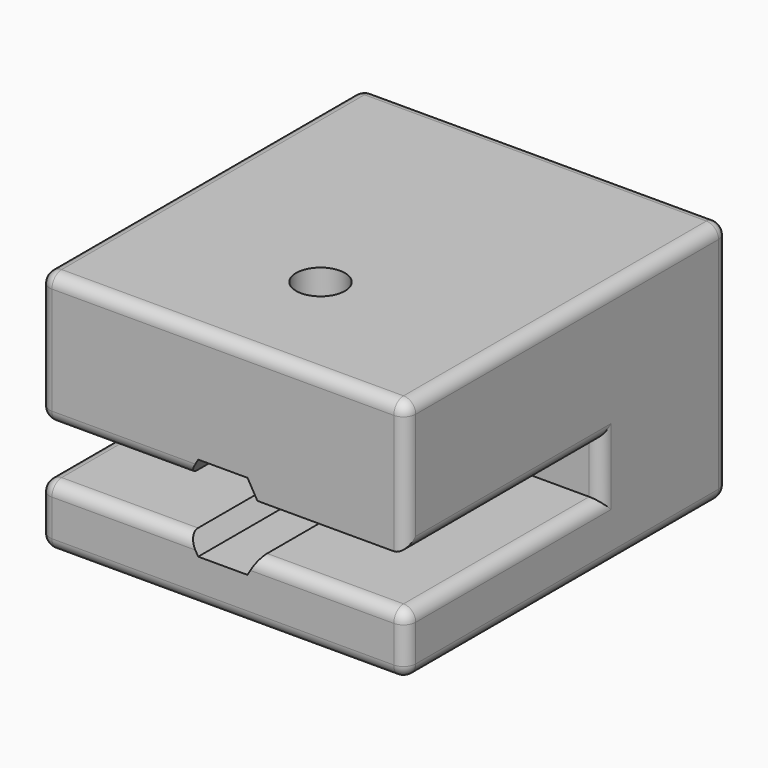
from build123d import *

# Parameters (mm, degrees)
F0_W          = 30
F0_H          = 33
F1_DEPTH      = 20
F2_W          = 20
F2_H          = 4.2
F3_DEPTH      = 30.001
F4_R          = 2
F5_DEPTH      = 5
F5_DEPTH_BACK = 20.001
F6_DEPTH      = 13.001
F7_R          = 2
F8_DEPTH      = 10.801
F9_DEPTH      = 3.5
F10_R         = 1


with BuildPart() as f1:
    # F0 (on Top) → F1 (new body)
    with BuildSketch(Plane.XY):
        Rectangle(F0_W, F0_H)
    extrude(amount=F1_DEPTH)

    # F2 (on face) → F3 (cut, through all)
    with BuildSketch(Plane.YZ.offset(15)):
        with Locations((-6.5, 7.1)):
            Rectangle(F2_W, F2_H)
    extrude(amount=-F3_DEPTH, mode=Mode.SUBTRACT)

    # F4 (on face) → F5 (cut, two sides)
    with BuildSketch(Plane.XZ.offset(-3.5)) as f5_sk:
        Polygon((-2.829016319, 9.2), (2.829016319, 9.2), (2.0207259422, 10.6), (-2.0207259422, 10.6), align=None)
        Polygon((-2.829016319, 5), (2.829016319, 5), (4.0414518843, 7.1), (2.829016319, 9.2), (-2.829016319, 9.2), (-4.0414518843, 7.1), align=None)
        with Locations((0, 7.1)):
            Circle(F4_R, mode=Mode.SUBTRACT)
        Polygon((-2.0207259422, 3.6), (2.0207259422, 3.6), (2.829016319, 5), (-2.829016319, 5), align=None)
    extrude(amount=-F5_DEPTH, mode=Mode.SUBTRACT)
    extrude(f5_sk.sketch, amount=F5_DEPTH_BACK, mode=Mode.SUBTRACT)

    # F6 (cut, through all): a face of the model
    f6_faces = [f1.faces().sort_by_distance(p)[0] for p in [
        (0, 3.5, 7.1),
    ]]
    extrude(f6_faces, amount=-F6_DEPTH, mode=Mode.SUBTRACT)

    # F7 (on face) → F8 (cut, through all)
    with BuildSketch(Plane(origin=(0, 0, 9.2), x_dir=(1, 0, 0), z_dir=(0, 0, -1))):
        with Locations((0, 6.5)):
            Circle(F7_R)
    extrude(amount=-F8_DEPTH, mode=Mode.SUBTRACT)

    # F7 (on face) → F9 (cut)
    with BuildSketch(Plane(origin=(0, 0, 9.2), x_dir=(1, 0, 0), z_dir=(0, 0, -1))):
        Polygon((-4.0414518843, 6.5), (-2.829016319, 4.4), (-2.829016319, 8.6), align=None)
        Polygon((-2.829016319, 8.6), (-2.829016319, 4.4), (-2.0207259422, 3), (2.0207259422, 3), (2.829016319, 4.4), (2.829016319, 8.6), (2.0207259422, 10), (-2.0207259422, 10), align=None)
        with Locations((0, 6.5)):
            Circle(F7_R, mode=Mode.SUBTRACT)
        Polygon((2.829016319, 8.6), (2.829016319, 4.4), (4.0414518843, 6.5), align=None)
    extrude(amount=-F9_DEPTH, mode=Mode.SUBTRACT)

    # F10
    f10_edges = [f1.edges().sort_by_distance(p)[0] for p in [
        (0, 16.5, 0),
        (15, 16.5, 10),
        (0, 16.5, 20),
        (-15, 16.5, 10),
        (-15, 0, 0),
        (0, -16.5, 0),
        (15, 0, 0),
        (-15, 0, 20),
        (0, -16.5, 20),
        (15, 0, 20),
        (-15, -16.5, 2.5),
        (-15, -16.5, 14.6),
        (15, -16.5, 2.5),
        (15, -16.5, 14.6),
        (15, -6.5, 9.2),
        (15, -6.5, 5),
        (8.914508, -16.5, 5),
        (-8.914508, -16.5, 5),
        (-8.914508, -16.5, 9.2),
        (-15, 3.5, 7.1),
        (-15, -6.5, 5),
        (-15, -6.5, 9.2),
        (15, 3.5, 7.1),
    ]]
    fillet(f10_edges, radius=F10_R)


solid = f1.part
